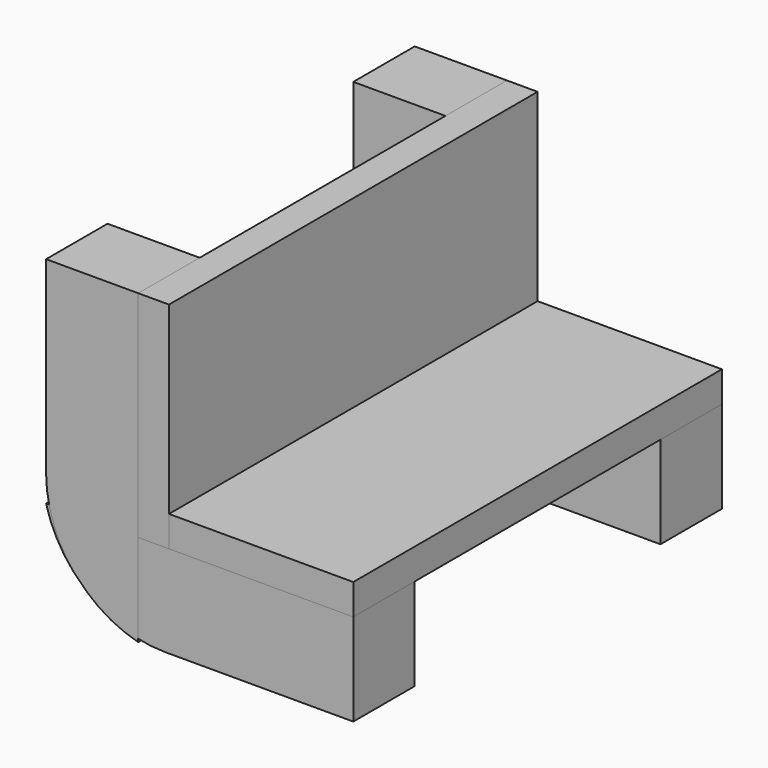
from build123d import *

# Parameters (mm, degrees)
F0_W          = 7
F0_H          = 2.5
F0_W_2        = 3
F1_DEPTH      = 3
F2_DEPTH      = 10
F3_W          = 7
F3_H          = 15
F4_DEPTH      = 1
F5_W          = 15
F5_H          = 7
F6_DEPTH      = 1
F7_T1_DEPTH   = 21.864916731
F8_T1_DEPTH   = 21.864916731
F8_2_T1_DEPTH = 21.864916731
F9_T1_DEPTH   = 21.864916731


# Not quite as in the source:
# - a fillet or chamfer that OpenCascade refuses, or shapes differently, is made with other operations: its cross-section is extruded or revolved along the edge and cut away or added


with BuildPart() as f1:
    # F0 (on Top) → F1 (new body)
    with BuildSketch(Plane.XY):
        with Locations((1.5, -6.25)):
            Rectangle(F0_W, F0_H)
        with Locations((-3.5, -6.25)):
            Rectangle(F0_W_2, F0_H)
    extrude(amount=F1_DEPTH)

    # F7: fillet of radius 4 on 1 edges, made by hand

    # F7_s2 → F7_t1 (cut)
    with BuildSketch(Plane.XZ.offset(-4.6824583655)):
        with BuildLine():
            ThreePointArc((-5, 3), (-3.5765063966, 0.8377223398), (-1.1270166538, 0))
            Line((-1.1270166538, 0), (-5, 0))
            Line((-5, 0), (-5, 3))
        make_face()
    extrude(amount=F7_T1_DEPTH, mode=Mode.SUBTRACT)


with BuildPart() as f1b:
    # F0 (on Top) → F1, piece 2 (new body)
    with BuildSketch(Plane.XY):
        with Locations((1.5, 6.25)):
            Rectangle(F0_W, F0_H)
        with Locations((-3.5, 6.25)):
            Rectangle(F0_W_2, F0_H)
    extrude(amount=F1_DEPTH)

    # F8: fillet of radius 4 on 1 edges, made by hand

    # F8_s2 → F8_t1 (cut)
    with BuildSketch(Plane.XZ.offset(-17.1824583655)):
        with BuildLine():
            ThreePointArc((-5, 3), (-3.5765063966, 0.8377223398), (-1.1270166538, 0))
            Line((-1.1270166538, 0), (-5, 0))
            Line((-5, 0), (-5, 3))
        make_face()
    extrude(amount=F8_T1_DEPTH, mode=Mode.SUBTRACT)


with BuildPart() as f2:
    # F0 (on Top) → F2 (new body)
    with BuildSketch(Plane.XY):
        with Locations((-3.5, -6.25)):
            Rectangle(F0_W_2, F0_H)
    extrude(amount=F2_DEPTH)

    # F8#2: fillet of radius 4 on 1 edges, made by hand

    # F8_2_s2 → F8_2_t1 (cut)
    with BuildSketch(Plane.XZ.offset(-4.6824583655)):
        with BuildLine():
            ThreePointArc((-5, 3.8729833462), (-4.1622776602, 1.4234936034), (-2, 0))
            Line((-2, 0), (-5, 0))
            Line((-5, 0), (-5, 3.8729833462))
        make_face()
    extrude(amount=F8_2_T1_DEPTH, mode=Mode.SUBTRACT)


with BuildPart() as f2b:
    # F0 (on Top) → F2, piece 2 (new body)
    with BuildSketch(Plane.XY):
        with Locations((-3.5, 6.25)):
            Rectangle(F0_W_2, F0_H)
    extrude(amount=F2_DEPTH)

    # F9: fillet of radius 4 on 1 edges, made by hand

    # F9_s2 → F9_t1 (cut)
    with BuildSketch(Plane.XZ.offset(-17.1824583655)):
        with BuildLine():
            ThreePointArc((-5, 3.8729833462), (-4.1622776602, 1.4234936034), (-2, 0))
            Line((-2, 0), (-5, 0))
            Line((-5, 0), (-5, 3.8729833462))
        make_face()
    extrude(amount=F9_T1_DEPTH, mode=Mode.SUBTRACT)


with BuildPart() as f4:
    # F3 (on face) → F4 (new body)
    with BuildSketch(Plane.XY.offset(3)):
        with Locations((1.5, 0)):
            Rectangle(F3_W, F3_H)
    extrude(amount=F4_DEPTH)


with BuildPart() as f6:
    # F5 (on face) → F6 (new body)
    with BuildSketch(Plane.YZ.offset(-2)):
        with Locations((0, 6.5)):
            Rectangle(F5_W, F5_H)
    extrude(amount=F6_DEPTH)


solid = Compound([f1.part, f1b.part, f2.part, f2b.part, f4.part, f6.part])
